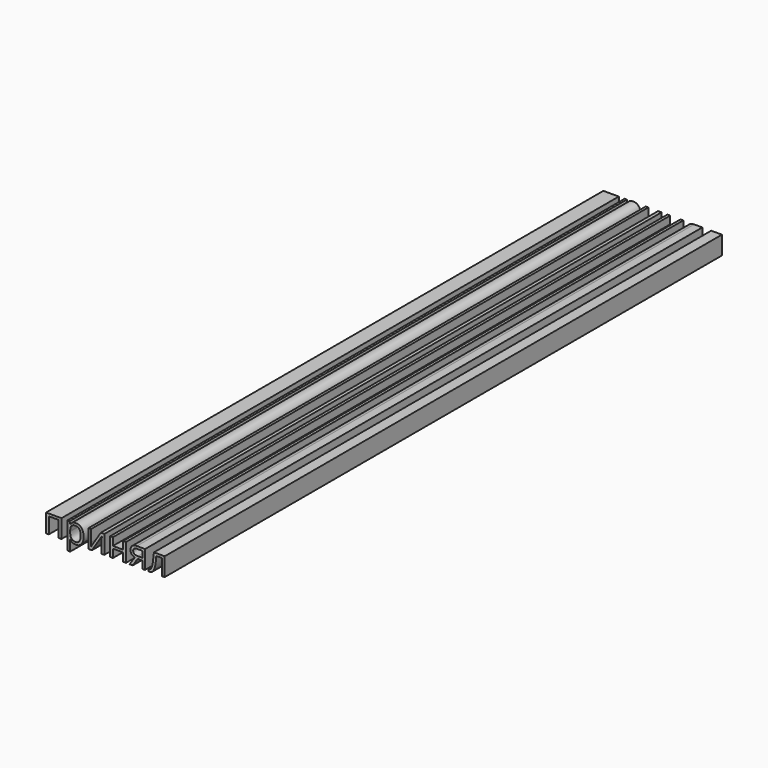
from build123d import *

# Parameters (mm, degrees)
F0_TEXT_SIZE = 31.2812626362
F1_DEPTH     = 635


# Not quite as in the source:
# - Text() gives the source's letters only with a copy of the font that has no kerning and outlines rounded to 1/6400 em; it was checked with that copy


with BuildPart() as f1:
    # F0 (on face) → F1 (new body)
    with BuildSketch(Plane.XZ):
        with Locations((-47.2008660436, 33.0503880978)):
            Text('принял', F0_TEXT_SIZE, font='Open Sans', text_align=(TextAlign.LEFT, TextAlign.BOTTOM))
    extrude(amount=F1_DEPTH)


solid = f1.part
